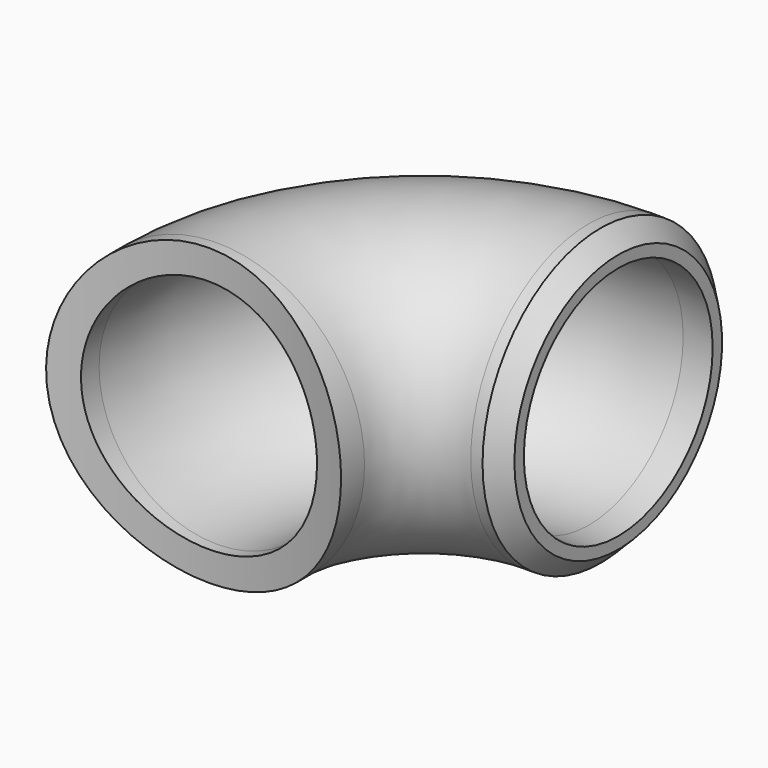
from build123d import *

# Parameters (mm, degrees)
F1_R     = 31.75
F1_R_2   = 25.399999693
F3_R     = 127
F4_DEPTH = 50.8
F5_SIZE  = 3.81


with BuildPart() as f2:
    # F2: sweep along a path in F0
    with BuildLine(Plane.XY) as f2_path:
        Line((0, 0), (0, 6.35))
        ThreePointArc((0, 6.35), (13.0191035763, 37.7808964237), (44.45, 50.8))
        Line((44.45, 50.8), (50.8, 50.8))
    # F1 (on Front) → F2 (sweep)
    with BuildSketch(Plane.XZ):
        Circle(F1_R)
        Circle(F1_R_2, mode=Mode.SUBTRACT)
    sweep(path=f2_path.line)

    # F3 (on Top) → F4 (cut, symmetric)
    with BuildSketch(Plane.XY):
        with Locations((0, -122.936)):
            Circle(F3_R)
    extrude(amount=F4_DEPTH, both=True, mode=Mode.SUBTRACT)

    # F5
    f5_edges = [f2.edges().sort_by_distance(p)[0] for p in [
        (50.8, 82.55, 0),
    ]]
    chamfer(f5_edges, length=F5_SIZE)


solid = f2.part
